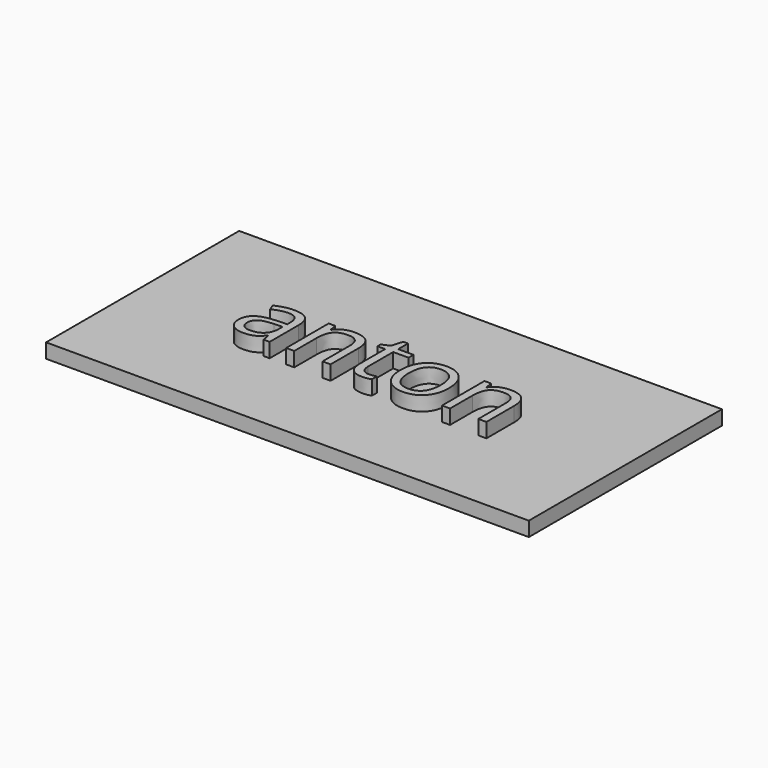
from build123d import *

# Parameters (mm, degrees)
F1_DEPTH     = 3
F2_TEXT_SIZE = 20.5469654045
F3_DEPTH     = 3


# Not quite as in the source:
# - Text() gives the source's letters only with a copy of the font that has no kerning and outlines rounded to 1/6400 em; it was checked with that copy


with BuildPart() as f1:
    # F0 (on Top) → F1 (new body)
    with BuildSketch(Plane.XY):
        Polygon((0, 50), (0, 0), (100, 0), (100, 50), (96.753830092, 50), align=None)
    extrude(amount=F1_DEPTH)

    # F2 (on face) → F3 (join)
    with BuildSketch(Plane.XY.offset(3)):
        with Locations((21.971645765, 18.2216502726)):
            Text('anton', F2_TEXT_SIZE, font='Open Sans', text_align=(TextAlign.LEFT, TextAlign.BOTTOM))
    extrude(amount=F3_DEPTH)


solid = f1.part
